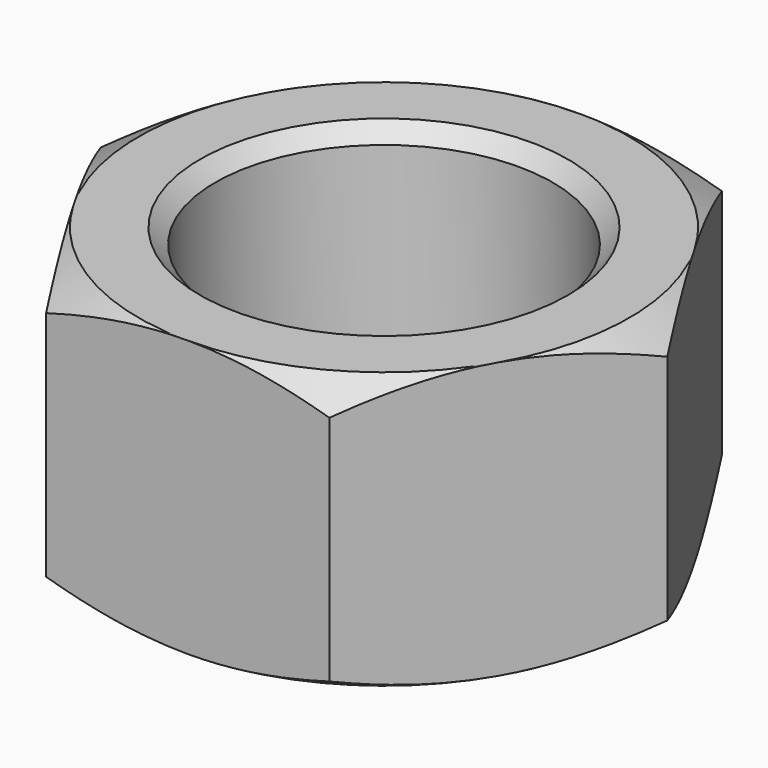
from build123d import *

# Parameters (mm, degrees)
F1_DEPTH = 18
F4_R     = 11
F5_DEPTH = 18.001
F6_SIZE  = 1


# Not quite as in the source:
# - a feature names something its author has since deleted; it is built from what else it names


with BuildPart() as f1:
    # F0 (on Top) → F1 (new body)
    with BuildSketch(Plane.XY):
        Polygon((18.4752086141, 0), (9.237604307, 16), (-9.237604307, 16), (-18.4752086141, 0), (-9.237604307, -16), (9.237604307, -16), align=None)
    extrude(amount=F1_DEPTH)

    # F2 (on Right) → F3 (revolve, cut)
    with BuildSketch(Plane.YZ):
        Polygon((-29.0477817086, 10.4668597182), (-16, 18), (-29.0477817086, 18), align=None)
        Polygon((-16, 0), (-29.0477817086, 7.5331402818), (-29.0477817086, 0), align=None)
    revolve(axis=Axis((0, 0, 10.077371262), (0, 0, 1)), mode=Mode.SUBTRACT)

    # F4 (on face) → F5 (cut, through all)
    with BuildSketch(Plane(origin=(0, 0, 0), x_dir=(1, 0, 0), z_dir=(0, 0, -1))):
        Circle(F4_R)
    extrude(amount=-F5_DEPTH, mode=Mode.SUBTRACT)

    # F6
    f6_edges = [f1.edges().sort_by_distance(p)[0] for p in [
        (-11, 0, 0),
        (-11, 0, 18),
    ]]
    chamfer(f6_edges, length=F6_SIZE)


solid = f1.part
